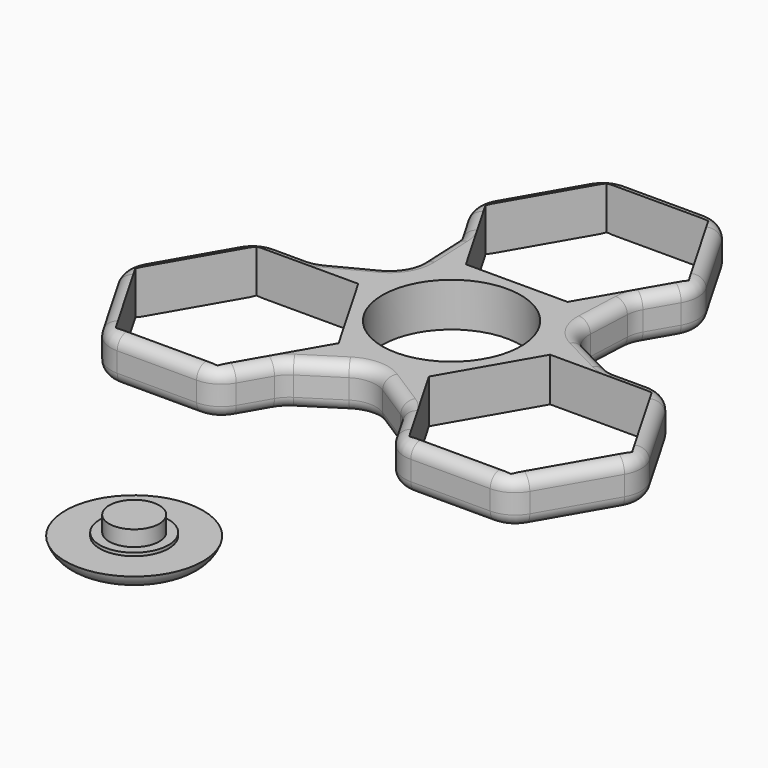
from build123d import *

# Parameters (mm, degrees)
F1_DEPTH       = 7
F2_R           = 5
F3_COUNT       = 3
F4_R           = 5
F5_R           = 11
F5_R_2         = 5.5
F6_DEPTH       = 2.5
F5_R_3         = 4
F7_DEPTH       = 3
F8_DEPTH       = 5.5
F10_T1_DEPTH   = 6.9965201323
F10_T3_DEPTH   = 6.9864388907
F10_T5_DEPTH   = 6.9965201323
F10_T7_DEPTH   = 5.1304731345
F10_T9_DEPTH   = 5.1287182285
F10_T11_DEPTH  = 12.7017059222
F10_T13_DEPTH  = 12.7017059222
F10_T15_DEPTH  = 12.7017059222
F10_T17_DEPTH  = 12.7017059222
F10_T19_DEPTH  = 12.7017059222
F10_T21_DEPTH  = 12.7017059222
F10_T23_DEPTH  = 5.1287182285
F10_T25_DEPTH  = 5.1304731345
F10_T27_DEPTH  = 6.9965201323
F10_T29_DEPTH  = 6.9864388907
F10_T31_DEPTH  = 6.9864388907
F10_T33_DEPTH  = 5.1304731345
F10_T35_DEPTH  = 5.1287182285
F10_T37_DEPTH  = 12.7017059222
F10_T39_DEPTH  = 12.7017059222
F10_T41_DEPTH  = 12.7017059222
F10_T44_ANGLE  = 65.096666036
F10_T46_ANGLE  = 27.4326894179
F10_T48_ANGLE  = 27.4706445461
F10_T50_ANGLE  = 60
F10_T52_ANGLE  = 60
F10_T54_ANGLE  = 60
F10_T56_ANGLE  = 60
F10_T58_ANGLE  = 60
F10_T60_ANGLE  = 60
F10_T62_ANGLE  = 60
F10_T64_ANGLE  = 60
F10_T66_ANGLE  = 27.4706445461
F10_T68_ANGLE  = 27.4326894179
F10_T70_ANGLE  = 65.096666036
F10_T72_ANGLE  = 65.096666036
F10_T74_ANGLE  = 27.4326894179
F10_T76_ANGLE  = 27.4706445461
F10_T78_ANGLE  = 60
F10_T80_ANGLE  = 60
F10_T82_ANGLE  = 60
F10_T84_ANGLE  = 60
F10_T86_ANGLE  = 65.096666036
F10_T88_ANGLE  = 27.4326894179
F10_T90_ANGLE  = 27.4706445461
F10_T92_ANGLE  = 60
F10_T94_ANGLE  = 60
F10_T96_ANGLE  = 60
F10_T98_ANGLE  = 60
F10_T100_ANGLE = 60
F10_T102_ANGLE = 60
F10_T104_ANGLE = 60
F10_T106_ANGLE = 60
F10_T108_ANGLE = 27.4706445461
F10_T110_ANGLE = 27.4326894179
F10_T112_ANGLE = 65.096666036
F10_T114_ANGLE = 65.096666036
F10_T116_ANGLE = 27.4326894179
F10_T118_ANGLE = 27.4706445461
F10_T120_ANGLE = 60
F10_T122_ANGLE = 60
F10_T124_ANGLE = 60
F10_T126_ANGLE = 60


# Not quite as in the source:
# - a fillet or chamfer that OpenCascade refuses, or shapes differently, is made with other operations: its cross-section is extruded or revolved along the edge and cut away or added


with BuildPart() as f1:
    # F0 (on Top) → F1 (new body)
    with BuildSketch(Plane.XY):
        with BuildLine():
            Line((13, 0), (11.075, 0))
            ThreePointArc((11.075, 0), (0, -11.075), (-11.075, 0))
            Line((-11.075, 0), (-13, 0))
            ThreePointArc((-13, 0), (0, -13), (13, 0))
        make_face()
        with BuildLine():
            ThreePointArc((-11.075, 0), (0, 11.075), (11.075, 0))
            Line((11.075, 0), (13, 0))
            ThreePointArc((13, 0), (11.3350959698, 6.3651865139), (6.7668308683, 11.1))
            Line((6.7668308683, 11.1), (-6.7668308683, 11.1))
            ThreePointArc((-6.7668308683, 11.1), (-11.3350959698, 6.3651865139), (-13, 0))
            Line((-13, 0), (-11.075, 0))
        make_face()
        with BuildLine():
            ThreePointArc((6.7668308683, 11.1), (11.3350959698, 6.3651865139), (13, 0))
            Line((13, 0), (13.0126777041, 0))
            Line((13.0126777041, 0), (13.8564064606, 19.1))
            Line((13.8564064606, 19.1), (9.237604307, 11.1))
            Line((9.237604307, 11.1), (6.7668308683, 11.1))
        make_face()
        with BuildLine():
            Line((-13.8564064606, 19.1), (-13, 0))
            ThreePointArc((-13, 0), (-11.3350959698, 6.3651865139), (-6.7668308683, 11.1))
            Line((-6.7668308683, 11.1), (-9.237604307, 11.1))
            Line((-9.237604307, 11.1), (-13.8564064606, 19.1))
        make_face()
        with BuildLine():
            ThreePointArc((-6.7668308683, 11.1), (0, 13), (6.7668308683, 11.1))
            Line((6.7668308683, 11.1), (9.237604307, 11.1))
            Line((9.237604307, 11.1), (13.8564064606, 19.1))
            Line((13.8564064606, 19.1), (18.4752086141, 27.1))
            Line((18.4752086141, 27.1), (9.237604307, 43.1))
            Line((9.237604307, 43.1), (-9.237604307, 43.1))
            Line((-9.237604307, 43.1), (-18.4752086141, 27.1))
            Line((-18.4752086141, 27.1), (-13.8564064606, 19.1))
            Line((-13.8564064606, 19.1), (-9.237604307, 11.1))
            Line((-9.237604307, 11.1), (-6.7668308683, 11.1))
        make_face()
        Polygon((16.2524100777, 27.1), (8.1262050388, 13.025), (-8.1262050388, 13.025), (-16.2524100777, 27.1), (-11.1141951775, 35.9996492673), (-8.1262050388, 41.175), (8.1262050388, 41.175), (11.1141951775, 35.9996492673), align=None, mode=Mode.SUBTRACT)
        with BuildLine():
            Line((-6.7668308683, 11.1), (6.7668308683, 11.1))
            ThreePointArc((6.7668308683, 11.1), (0, 13), (-6.7668308683, 11.1))
        make_face()
    extrude(amount=F1_DEPTH)

    # F2
    f2_edges = [f1.edges().sort_by_distance(p)[0] for p in [
        (-18.475209, 27.1, 3.5),
        (-9.237604, 43.1, 3.5),
        (9.237604, 43.1, 3.5),
        (18.475209, 27.1, 3.5),
        (13.856406, 19.1, 3.5),
        (-13.856406, 19.1, 3.5),
    ]]
    fillet(f2_edges, radius=F2_R)

    # F3: F1 ×3 about axis
    f3_axis = Axis((0, 0, 0), (0, 0, -1))


with BuildPart() as f1_1:
    add(f1.part)
    for i in range(1, F3_COUNT):
        add(f1.part.rotate(f3_axis, i * 360 / F3_COUNT))

    # F4
    f4_edges = [f1_1.edges().sort_by_distance(p)[0] for p in [
        (-13.345851, 7.713337, 3.5),
        (13.352872, 7.701177, 3.5),
        (-0.007021, -15.414515, 3.5),
    ]]
    fillet(f4_edges, radius=F4_R)

    # F10: fillet of radius 1.925 on 84 edges, made by hand

    # F10_s2 → F10_t1 (cut)
    with BuildSketch(Plane(origin=(0.5063723559, 11.4630583874, 0), x_dir=(0, 0, 1), z_dir=(0.0441312433, 0.9990257421, 0))):
        with BuildLine():
            ThreePointArc((5.075, 13), (6.4361805538, 12.4361805538), (7, 11.075))
            Line((7, 11.075), (7, 13))
            Line((7, 13), (5.075, 13))
        make_face()
        with BuildLine():
            ThreePointArc((0, 11.075), (0.5638194462, 12.4361805538), (1.925, 13))
            Line((1.925, 13), (0, 13))
            Line((0, 13), (0, 11.075))
        make_face()
    extrude(amount=F10_T1_DEPTH, mode=Mode.SUBTRACT)

    # F10_s4 → F10_t3 (cut)
    with BuildSketch(Plane(origin=(-15.5751419663, -9.9482027869, 0), x_dir=(0, 0, 1), z_dir=(0.8427596491, 0.5382900463, 0))):
        with BuildLine():
            ThreePointArc((0, 11.0619517506), (0.5638194462, 12.4231323044), (1.925, 12.9869517506))
            Line((1.925, 12.9869517506), (0, 12.9869517506))
            Line((0, 12.9869517506), (0, 11.0619517506))
        make_face()
        with BuildLine():
            ThreePointArc((5.075, 12.9869517506), (6.4361805538, 12.4231323044), (7, 11.0619517506))
            Line((7, 11.0619517506), (7, 12.9869517506))
            Line((7, 12.9869517506), (5.075, 12.9869517506))
        make_face()
    extrude(amount=F10_T3_DEPTH, mode=Mode.SUBTRACT)

    # F10_s6 → F10_t5 (cut)
    with BuildSketch(Plane(origin=(9.6741135906, -6.1700605177, 0), x_dir=(0, 0, 1), z_dir=(0.84311605, -0.5377316488, 0))):
        with BuildLine():
            ThreePointArc((0, 11.075), (0.5638194462, 12.4361805538), (1.925, 13))
            Line((1.925, 13), (0, 13))
            Line((0, 13), (0, 11.075))
        make_face()
        with BuildLine():
            ThreePointArc((5.075, 13), (6.4361805538, 12.4361805538), (7, 11.075))
            Line((7, 11.075), (7, 13))
            Line((7, 13), (5.075, 13))
        make_face()
    extrude(amount=F10_T5_DEPTH, mode=Mode.SUBTRACT)

    # F10_s8 → F10_t7 (cut)
    with BuildSketch(Plane(origin=(-14.9100707018, -25.825, 0), x_dir=(0, 0, 1), z_dir=(0.5, 0.8660254038, 0))):
        with BuildLine():
            ThreePointArc((0, 0.525), (0.5638194462, 1.8861805538), (1.925, 2.45))
            Line((1.925, 2.45), (0, 2.45))
            Line((0, 2.45), (0, 0.525))
        make_face()
        with BuildLine():
            ThreePointArc((5.075, 2.45), (6.4361805538, 1.8861805538), (7, 0.525))
            Line((7, 0.525), (7, 2.45))
            Line((7, 2.45), (5.075, 2.45))
        make_face()
    extrude(amount=F10_T7_DEPTH, mode=Mode.SUBTRACT)

    # F10_s10 → F10_t9 (cut)
    with BuildSketch(Plane(origin=(12.3457115876, -21.3833997253, 0), x_dir=(0, 0, 1), z_dir=(0.5, -0.8660254038, 0))):
        with BuildLine():
            ThreePointArc((0, 0.525), (0.5638194462, 1.8861805538), (1.925, 2.45))
            Line((1.925, 2.45), (0, 2.45))
            Line((0, 2.45), (0, 0.525))
        make_face()
        with BuildLine():
            ThreePointArc((5.075, 2.45), (6.4361805538, 1.8861805538), (7, 0.525))
            Line((7, 0.525), (7, 2.45))
            Line((7, 2.45), (5.075, 2.45))
        make_face()
    extrude(amount=F10_T9_DEPTH, mode=Mode.SUBTRACT)

    # F10_s12 → F10_t11 (cut)
    with BuildSketch(Plane.YZ.offset(-29.8201414036)):
        with BuildLine():
            ThreePointArc((-27.625, 0), (-28.9861805538, 0.5638194462), (-29.55, 1.925))
            Line((-29.55, 1.925), (-29.55, 0))
            Line((-29.55, 0), (-27.625, 0))
        make_face()
        with BuildLine():
            ThreePointArc((-29.55, 5.075), (-28.9861805538, 6.4361805538), (-27.625, 7))
            Line((-27.625, 7), (-29.55, 7))
            Line((-29.55, 7), (-29.55, 5.075))
        make_face()
    extrude(amount=F10_T11_DEPTH, mode=Mode.SUBTRACT)

    # F10_s14 → F10_t13 (cut)
    with BuildSketch(Plane.YZ.offset(17.1184354815)):
        with BuildLine():
            ThreePointArc((-27.625, 0), (-28.9861805538, 0.5638194462), (-29.55, 1.925))
            Line((-29.55, 1.925), (-29.55, 0))
            Line((-29.55, 0), (-27.625, 0))
        make_face()
        with BuildLine():
            ThreePointArc((-29.55, 5.075), (-28.9861805538, 6.4361805538), (-27.625, 7))
            Line((-27.625, 7), (-29.55, 7))
            Line((-29.55, 7), (-29.55, 5.075))
        make_face()
    extrude(amount=F10_T13_DEPTH, mode=Mode.SUBTRACT)

    # F10_s16 → F10_t15 (cut)
    with BuildSketch(Plane(origin=(-3.1754264805, 5.5, 0), x_dir=(0, 0, 1), z_dir=(0.5, -0.8660254038, 0))):
        with BuildLine():
            ThreePointArc((0, 41.175), (0.5638194462, 42.5361805538), (1.925, 43.1))
            Line((1.925, 43.1), (0, 43.1))
            Line((0, 43.1), (0, 41.175))
        make_face()
        with BuildLine():
            ThreePointArc((5.075, 43.1), (6.4361805538, 42.5361805538), (7, 41.175))
            Line((7, 41.175), (7, 43.1))
            Line((7, 43.1), (5.075, 43.1))
        make_face()
    extrude(amount=F10_T15_DEPTH, mode=Mode.SUBTRACT)

    # F10_s18 → F10_t17 (cut)
    with BuildSketch(Plane(origin=(-3.1754264805, -5.5, 0), x_dir=(0, 0, 1), z_dir=(0.5, 0.8660254038, 0))):
        with BuildLine():
            ThreePointArc((0, 41.175), (0.5638194462, 42.5361805538), (1.925, 43.1))
            Line((1.925, 43.1), (0, 43.1))
            Line((0, 43.1), (0, 41.175))
        make_face()
        with BuildLine():
            ThreePointArc((5.075, 43.1), (6.4361805538, 42.5361805538), (7, 41.175))
            Line((7, 41.175), (7, 43.1))
            Line((7, 43.1), (5.075, 43.1))
        make_face()
    extrude(amount=F10_T17_DEPTH, mode=Mode.SUBTRACT)

    # F10_s20 → F10_t19 (cut)
    with BuildSketch(Plane(origin=(-8.5592177407, -14.825, 0), x_dir=(0, 0, 1), z_dir=(-0.5, -0.8660254038, 0))):
        with BuildLine():
            ThreePointArc((0, 27.625), (0.5638194462, 28.9861805538), (1.925, 29.55))
            Line((1.925, 29.55), (0, 29.55))
            Line((0, 29.55), (0, 27.625))
        make_face()
        with BuildLine():
            ThreePointArc((5.075, 29.55), (6.4361805538, 28.9861805538), (7, 27.625))
            Line((7, 27.625), (7, 29.55))
            Line((7, 29.55), (5.075, 29.55))
        make_face()
    extrude(amount=F10_T19_DEPTH, mode=Mode.SUBTRACT)

    # F10_s22 → F10_t21 (cut)
    with BuildSketch(Plane(origin=(14.9100707018, -25.825, 0), x_dir=(0, 0, 1), z_dir=(-0.5, 0.8660254038, 0))):
        with BuildLine():
            ThreePointArc((0, 27.625), (0.5638194462, 28.9861805538), (1.925, 29.55))
            Line((1.925, 29.55), (0, 29.55))
            Line((0, 29.55), (0, 27.625))
        make_face()
        with BuildLine():
            ThreePointArc((5.075, 29.55), (6.4361805538, 28.9861805538), (7, 27.625))
            Line((7, 27.625), (7, 29.55))
            Line((7, 29.55), (5.075, 29.55))
        make_face()
    extrude(amount=F10_T21_DEPTH, mode=Mode.SUBTRACT)

    # F10_s24 → F10_t23 (cut)
    with BuildSketch(Plane.YZ.offset(-29.8201414036)):
        with BuildLine():
            ThreePointArc((0.525, 0), (1.8861805538, 0.5638194462), (2.45, 1.925))
            Line((2.45, 1.925), (2.45, 0))
            Line((2.45, 0), (0.525, 0))
        make_face()
        with BuildLine():
            ThreePointArc((2.45, 5.075), (1.8861805538, 6.4361805538), (0.525, 7))
            Line((0.525, 7), (2.45, 7))
            Line((2.45, 7), (2.45, 5.075))
        make_face()
    extrude(amount=F10_T23_DEPTH, mode=Mode.SUBTRACT)

    # F10_s26 → F10_t25 (cut)
    with BuildSketch(Plane.YZ.offset(24.6896682691)):
        with BuildLine():
            ThreePointArc((0.525, 0), (1.8861805538, 0.5638194462), (2.45, 1.925))
            Line((2.45, 1.925), (2.45, 0))
            Line((2.45, 0), (0.525, 0))
        make_face()
        with BuildLine():
            ThreePointArc((2.45, 5.075), (1.8861805538, 6.4361805538), (0.525, 7))
            Line((0.525, 7), (2.45, 7))
            Line((2.45, 7), (2.45, 5.075))
        make_face()
    extrude(amount=F10_T25_DEPTH, mode=Mode.SUBTRACT)

    # F10_s28 → F10_t27 (cut)
    with BuildSketch(Plane(origin=(-10.1804859465, -5.2929978697, 0), x_dir=(0, 0, 1), z_dir=(-0.8872472933, -0.4612940932, 0))):
        with BuildLine():
            ThreePointArc((0, 11.075), (0.5638194462, 12.4361805538), (1.925, 13))
            Line((1.925, 13), (0, 13))
            Line((0, 13), (0, 11.075))
        make_face()
        with BuildLine():
            ThreePointArc((5.075, 13), (6.4361805538, 12.4361805538), (7, 11.075))
            Line((7, 11.075), (7, 13))
            Line((7, 13), (5.075, 13))
        make_face()
    extrude(amount=F10_T27_DEPTH, mode=Mode.SUBTRACT)

    # F10_s30 → F10_t29 (cut)
    with BuildSketch(Plane(origin=(16.4029673186, -8.5143672169, 0), x_dir=(0, 0, 1), z_dir=(-0.8875526792, 0.4607062422, 0))):
        with BuildLine():
            ThreePointArc((0, 11.0619517506), (0.5638194462, 12.4231323044), (1.925, 12.9869517506))
            Line((1.925, 12.9869517506), (0, 12.9869517506))
            Line((0, 12.9869517506), (0, 11.0619517506))
        make_face()
        with BuildLine():
            ThreePointArc((5.075, 12.9869517506), (6.4361805538, 12.4231323044), (7, 11.0619517506))
            Line((7, 11.0619517506), (7, 12.9869517506))
            Line((7, 12.9869517506), (5.075, 12.9869517506))
        make_face()
    extrude(amount=F10_T29_DEPTH, mode=Mode.SUBTRACT)

    # F10_s32 → F10_t31 (cut)
    with BuildSketch(Plane(origin=(-0.8278253523, 18.4625700038, 0), x_dir=(0, 0, 1), z_dir=(0.0447930301, -0.9989962885, 0))):
        with BuildLine():
            ThreePointArc((0, 11.0619517506), (0.5638194462, 12.4231323044), (1.925, 12.9869517506))
            Line((1.925, 12.9869517506), (0, 12.9869517506))
            Line((0, 12.9869517506), (0, 11.0619517506))
        make_face()
        with BuildLine():
            ThreePointArc((5.075, 12.9869517506), (6.4361805538, 12.4231323044), (7, 11.0619517506))
            Line((7, 11.0619517506), (7, 12.9869517506))
            Line((7, 12.9869517506), (5.075, 12.9869517506))
        make_face()
    extrude(amount=F10_T31_DEPTH, mode=Mode.SUBTRACT)

    # F10_s34 → F10_t33 (cut)
    with BuildSketch(Plane(origin=(-14.9100707018, 25.825, 0), x_dir=(0, 0, 1), z_dir=(0.5, -0.8660254038, 0))):
        with BuildLine():
            ThreePointArc((0, 0.525), (0.5638194462, 1.8861805538), (1.925, 2.45))
            Line((1.925, 2.45), (0, 2.45))
            Line((0, 2.45), (0, 0.525))
        make_face()
        with BuildLine():
            ThreePointArc((5.075, 2.45), (6.4361805538, 1.8861805538), (7, 0.525))
            Line((7, 0.525), (7, 2.45))
            Line((7, 2.45), (5.075, 2.45))
        make_face()
    extrude(amount=F10_T33_DEPTH, mode=Mode.SUBTRACT)

    # F10_s36 → F10_t35 (cut)
    with BuildSketch(Plane(origin=(12.3457115876, 21.3833997253, 0), x_dir=(0, 0, 1), z_dir=(0.5, 0.8660254038, 0))):
        with BuildLine():
            ThreePointArc((0, 0.525), (0.5638194462, 1.8861805538), (1.925, 2.45))
            Line((1.925, 2.45), (0, 2.45))
            Line((0, 2.45), (0, 0.525))
        make_face()
        with BuildLine():
            ThreePointArc((5.075, 2.45), (6.4361805538, 1.8861805538), (7, 0.525))
            Line((7, 0.525), (7, 2.45))
            Line((7, 2.45), (5.075, 2.45))
        make_face()
    extrude(amount=F10_T35_DEPTH, mode=Mode.SUBTRACT)

    # F10_s38 → F10_t37 (cut)
    with BuildSketch(Plane(origin=(14.9100707018, 25.825, 0), x_dir=(0, 0, 1), z_dir=(-0.5, -0.8660254038, 0))):
        with BuildLine():
            ThreePointArc((0, 27.625), (0.5638194462, 28.9861805538), (1.925, 29.55))
            Line((1.925, 29.55), (0, 29.55))
            Line((0, 29.55), (0, 27.625))
        make_face()
        with BuildLine():
            ThreePointArc((5.075, 29.55), (6.4361805538, 28.9861805538), (7, 27.625))
            Line((7, 27.625), (7, 29.55))
            Line((7, 29.55), (5.075, 29.55))
        make_face()
    extrude(amount=F10_T37_DEPTH, mode=Mode.SUBTRACT)

    # F10_s40 → F10_t39 (cut)
    with BuildSketch(Plane(origin=(-8.5592177407, 14.825, 0), x_dir=(0, 0, 1), z_dir=(-0.5, 0.8660254038, 0))):
        with BuildLine():
            ThreePointArc((0, 27.625), (0.5638194462, 28.9861805538), (1.925, 29.55))
            Line((1.925, 29.55), (0, 29.55))
            Line((0, 29.55), (0, 27.625))
        make_face()
        with BuildLine():
            ThreePointArc((5.075, 29.55), (6.4361805538, 28.9861805538), (7, 27.625))
            Line((7, 27.625), (7, 29.55))
            Line((7, 29.55), (5.075, 29.55))
        make_face()
    extrude(amount=F10_T39_DEPTH, mode=Mode.SUBTRACT)

    # F10_s42 → F10_t41 (cut)
    with BuildSketch(Plane.YZ.offset(-6.3508529611)):
        with BuildLine():
            ThreePointArc((41.175, 0), (42.5361805538, 0.5638194462), (43.1, 1.925))
            Line((43.1, 1.925), (43.1, 0))
            Line((43.1, 0), (41.175, 0))
        make_face()
        with BuildLine():
            ThreePointArc((43.1, 5.075), (42.5361805538, 6.4361805538), (41.175, 7))
            Line((41.175, 7), (43.1, 7))
            Line((43.1, 7), (43.1, 5.075))
        make_face()
    extrude(amount=F10_T41_DEPTH, mode=Mode.SUBTRACT)

    # F10_s43 → F10_t44 (revolve, cut)
    with BuildSketch(Plane(origin=(9.6741135906, -6.1700605177, 0), x_dir=(0, 0, 1), z_dir=(0.84311605, -0.5377316488, 0))):
        with BuildLine():
            ThreePointArc((0, 11.075), (0.5638194462, 12.4361805538), (1.925, 13))
            Line((1.925, 13), (0, 13))
            Line((0, 13), (0, 11.075))
        make_face()
    revolve(axis=Axis((-0.0050560886, -21.3461494184, 0), (0, 0, 1)), revolution_arc=F10_T44_ANGLE, mode=Mode.SUBTRACT)

    # F10_s45 → F10_t46 (revolve, cut)
    with BuildSketch(Plane(origin=(-12.3448341345, -21.3818799321, 0), x_dir=(0, 0, 1), z_dir=(-0.5, -0.8660254038, 0))):
        with BuildLine():
            ThreePointArc((0, -0.525), (0.5638194462, -1.8861805538), (1.925, -2.45))
            Line((1.925, -2.45), (0, -2.45))
            Line((0, -2.45), (0, -0.525))
        make_face()
    revolve(axis=Axis((-5.8929448764, -25.1068799321, 0), (0, 0, -1)), revolution_arc=F10_T46_ANGLE, mode=Mode.SUBTRACT)

    # F10_s47 → F10_t48 (revolve, cut)
    with BuildSketch(Plane(origin=(15.5729920086, -9.9323108246, 0), x_dir=(0, 0, 1), z_dir=(-0.84311605, 0.5377316488, 0))):
        with BuildLine():
            ThreePointArc((0, -11.075), (0.5638194462, -12.4361805538), (1.925, -13))
            Line((1.925, -13), (0, -13))
            Line((0, -13), (0, -11.075))
        make_face()
    revolve(axis=Axis((5.8938223294, -25.1083997253, 0), (0, 0, -1)), revolution_arc=F10_T48_ANGLE, mode=Mode.SUBTRACT)

    # F10_s49 → F10_t50 (revolve, cut)
    with BuildSketch(Plane.YZ.offset(-17.1184354815)):
        with BuildLine():
            ThreePointArc((-27.625, 0), (-28.9861805538, 0.5638194462), (-29.55, 1.925))
            Line((-29.55, 1.925), (-29.55, 0))
            Line((-29.55, 0), (-27.625, 0))
        make_face()
    revolve(axis=Axis((-17.1184354815, -24.55, 0), (0, 0, 1)), revolution_arc=F10_T50_ANGLE, mode=Mode.SUBTRACT)

    # F10_s51 → F10_t52 (revolve, cut)
    with BuildSketch(Plane(origin=(14.9100707018, -25.825, 0), x_dir=(0, 0, 1), z_dir=(-0.5, 0.8660254038, 0))):
        with BuildLine():
            ThreePointArc((0, -0.525), (0.5638194462, -1.8861805538), (1.925, -2.45))
            Line((1.925, -2.45), (0, -2.45))
            Line((0, -2.45), (0, -0.525))
        make_face()
    revolve(axis=Axis((17.1184354815, -24.55, 0), (0, 0, 1)), revolution_arc=F10_T52_ANGLE, mode=Mode.SUBTRACT)

    # F10_s53 → F10_t54 (revolve, cut)
    with BuildSketch(Plane(origin=(3.1754264805, -5.5, 0), x_dir=(0, 0, 1), z_dir=(-0.5, 0.8660254038, 0))):
        with BuildLine():
            ThreePointArc((0, -41.175), (0.5638194462, -42.5361805538), (1.925, -43.1))
            Line((1.925, -43.1), (0, -43.1))
            Line((0, -43.1), (0, -41.175))
        make_face()
    revolve(axis=Axis((-29.8201414036, -24.55, 0), (0, 0, 1)), revolution_arc=F10_T54_ANGLE, mode=Mode.SUBTRACT)

    # F10_s55 → F10_t56 (revolve, cut)
    with BuildSketch(Plane.YZ.offset(29.8201414036)):
        with BuildLine():
            ThreePointArc((-27.625, 0), (-28.9861805538, 0.5638194462), (-29.55, 1.925))
            Line((-29.55, 1.925), (-29.55, 0))
            Line((-29.55, 0), (-27.625, 0))
        make_face()
    revolve(axis=Axis((29.8201414036, -24.55, 0), (0, 0, 1)), revolution_arc=F10_T56_ANGLE, mode=Mode.SUBTRACT)

    # F10_s57 → F10_t58 (revolve, cut)
    with BuildSketch(Plane(origin=(-14.9100707018, -25.825, 0), x_dir=(0, 0, 1), z_dir=(0.5, 0.8660254038, 0))):
        with BuildLine():
            ThreePointArc((0, -27.625), (0.5638194462, -28.9861805538), (1.925, -29.55))
            Line((1.925, -29.55), (0, -29.55))
            Line((0, -29.55), (0, -27.625))
        make_face()
    revolve(axis=Axis((-36.1709943647, -13.55, 0), (0, 0, 1)), revolution_arc=F10_T58_ANGLE, mode=Mode.SUBTRACT)

    # F10_s59 → F10_t60 (revolve, cut)
    with BuildSketch(Plane(origin=(3.1754264805, 5.5, 0), x_dir=(0, 0, 1), z_dir=(-0.5, -0.8660254038, 0))):
        with BuildLine():
            ThreePointArc((0, -41.175), (0.5638194462, -42.5361805538), (1.925, -43.1))
            Line((1.925, -43.1), (0, -43.1))
            Line((0, -43.1), (0, -41.175))
        make_face()
    revolve(axis=Axis((36.1709943647, -13.55, 0), (0, 0, 1)), revolution_arc=F10_T60_ANGLE, mode=Mode.SUBTRACT)

    # F10_s61 → F10_t62 (revolve, cut)
    with BuildSketch(Plane.YZ.offset(-29.8201414036)):
        with BuildLine():
            ThreePointArc((0.525, 0), (1.8861805538, 0.5638194462), (2.45, 1.925))
            Line((2.45, 1.925), (2.45, 0))
            Line((2.45, 0), (0.525, 0))
        make_face()
    revolve(axis=Axis((-29.8201414036, -2.55, 0), (0, 0, 1)), revolution_arc=F10_T62_ANGLE, mode=Mode.SUBTRACT)

    # F10_s63 → F10_t64 (revolve, cut)
    with BuildSketch(Plane(origin=(8.5592177407, -14.825, 0), x_dir=(0, 0, 1), z_dir=(0.5, -0.8660254038, 0))):
        with BuildLine():
            ThreePointArc((0, -27.625), (0.5638194462, -28.9861805538), (1.925, -29.55))
            Line((1.925, -29.55), (0, -29.55))
            Line((0, -29.55), (0, -27.625))
        make_face()
    revolve(axis=Axis((29.8201414036, -2.55, 0), (0, 0, 1)), revolution_arc=F10_T64_ANGLE, mode=Mode.SUBTRACT)

    # F10_s65 → F10_t66 (revolve, cut)
    with BuildSketch(Plane(origin=(-16.3881294967, -8.5204512801, 0), x_dir=(0, 0, 1), z_dir=(0.8872472933, 0.4612940932, 0))):
        with BuildLine():
            ThreePointArc((0, -11.075), (0.5638194462, -12.4361805538), (1.925, -13))
            Line((1.925, -13), (0, -13))
            Line((0, -13), (0, -11.075))
        make_face()
    revolve(axis=Axis((-24.6914231752, 7.45, 0), (0, 0, -1)), revolution_arc=F10_T66_ANGLE, mode=Mode.SUBTRACT)

    # F10_s67 → F10_t68 (revolve, cut)
    with BuildSketch(Plane.YZ.offset(24.6896682691)):
        with BuildLine():
            ThreePointArc((0.525, 0), (1.8861805538, 0.5638194462), (2.45, 1.925))
            Line((2.45, 1.925), (2.45, 0))
            Line((2.45, 0), (0.525, 0))
        make_face()
    revolve(axis=Axis((24.6896682691, 7.45, 0), (0, 0, -1)), revolution_arc=F10_T68_ANGLE, mode=Mode.SUBTRACT)

    # F10_s69 → F10_t70 (revolve, cut)
    with BuildSketch(Plane(origin=(-10.1804859465, -5.2929978697, 0), x_dir=(0, 0, 1), z_dir=(-0.8872472933, -0.4612940932, 0))):
        with BuildLine():
            ThreePointArc((0, 11.075), (0.5638194462, 12.4361805538), (1.925, 13))
            Line((1.925, 13), (0, 13))
            Line((0, 13), (0, 11.075))
        make_face()
    revolve(axis=Axis((-18.483779625, 10.6774534104, 0), (0, 0, 1)), revolution_arc=F10_T70_ANGLE, mode=Mode.SUBTRACT)

    # F10_s71 → F10_t72 (revolve, cut)
    with BuildSketch(Plane(origin=(0.5063723559, 11.4630583874, 0), x_dir=(0, 0, 1), z_dir=(0.0441312433, 0.9990257421, 0))):
        with BuildLine():
            ThreePointArc((0, 11.075), (0.5638194462, 12.4361805538), (1.925, 13))
            Line((1.925, 13), (0, 13))
            Line((0, 13), (0, 11.075))
        make_face()
    revolve(axis=Axis((18.4888357136, 10.668696008, 0), (0, 0, 1)), revolution_arc=F10_T72_ANGLE, mode=Mode.SUBTRACT)

    # F10_s73 → F10_t74 (revolve, cut)
    with BuildSketch(Plane(origin=(-12.3448341345, 21.3818799321, 0), x_dir=(0, 0, 1), z_dir=(-0.5, 0.8660254038, 0))):
        with BuildLine():
            ThreePointArc((0, -0.525), (0.5638194462, -1.8861805538), (1.925, -2.45))
            Line((1.925, -2.45), (0, -2.45))
            Line((0, -2.45), (0, -0.525))
        make_face()
    revolve(axis=Axis((-18.7967233927, 17.6568799321, 0), (0, 0, -1)), revolution_arc=F10_T74_ANGLE, mode=Mode.SUBTRACT)

    # F10_s75 → F10_t76 (revolve, cut)
    with BuildSketch(Plane(origin=(0.8151374881, 18.4527621047, 0), x_dir=(0, 0, 1), z_dir=(-0.0441312433, -0.9990257421, 0))):
        with BuildLine():
            ThreePointArc((0, -11.075), (0.5638194462, -12.4361805538), (1.925, -13))
            Line((1.925, -13), (0, -13))
            Line((0, -13), (0, -11.075))
        make_face()
    revolve(axis=Axis((18.7976008458, 17.6583997253, 0), (0, 0, -1)), revolution_arc=F10_T76_ANGLE, mode=Mode.SUBTRACT)

    # F10_s77 → F10_t78 (revolve, cut)
    with BuildSketch(Plane(origin=(8.5592177407, 14.825, 0), x_dir=(0, 0, 1), z_dir=(0.5, 0.8660254038, 0))):
        with BuildLine():
            ThreePointArc((0, -27.625), (0.5638194462, -28.9861805538), (1.925, -29.55))
            Line((1.925, -29.55), (0, -29.55))
            Line((0, -29.55), (0, -27.625))
        make_face()
    revolve(axis=Axis((-12.7017059222, 27.1, 0), (0, 0, 1)), revolution_arc=F10_T78_ANGLE, mode=Mode.SUBTRACT)

    # F10_s79 → F10_t80 (revolve, cut)
    with BuildSketch(Plane(origin=(14.9100707018, 25.825, 0), x_dir=(0, 0, 1), z_dir=(-0.5, -0.8660254038, 0))):
        with BuildLine():
            ThreePointArc((0, -0.525), (0.5638194462, -1.8861805538), (1.925, -2.45))
            Line((1.925, -2.45), (0, -2.45))
            Line((0, -2.45), (0, -0.525))
        make_face()
    revolve(axis=Axis((12.7017059222, 27.1, 0), (0, 0, 1)), revolution_arc=F10_T80_ANGLE, mode=Mode.SUBTRACT)

    # F10_s81 → F10_t82 (revolve, cut)
    with BuildSketch(Plane.YZ.offset(-6.3508529611)):
        with BuildLine():
            ThreePointArc((41.175, 0), (42.5361805538, 0.5638194462), (43.1, 1.925))
            Line((43.1, 1.925), (43.1, 0))
            Line((43.1, 0), (41.175, 0))
        make_face()
    revolve(axis=Axis((-6.3508529611, 38.1, 0), (0, 0, 1)), revolution_arc=F10_T82_ANGLE, mode=Mode.SUBTRACT)

    # F10_s83 → F10_t84 (revolve, cut)
    with BuildSketch(Plane(origin=(-14.9100707018, 25.825, 0), x_dir=(0, 0, 1), z_dir=(0.5, -0.8660254038, 0))):
        with BuildLine():
            ThreePointArc((0, -27.625), (0.5638194462, -28.9861805538), (1.925, -29.55))
            Line((1.925, -29.55), (0, -29.55))
            Line((0, -29.55), (0, -27.625))
        make_face()
    revolve(axis=Axis((6.3508529611, 38.1, 0), (0, 0, 1)), revolution_arc=F10_T84_ANGLE, mode=Mode.SUBTRACT)

    # F10_s85 → F10_t86 (revolve, cut)
    with BuildSketch(Plane(origin=(9.6741135906, -6.1700605177, 0), x_dir=(0, 0, 1), z_dir=(0.84311605, -0.5377316488, 0))):
        with BuildLine():
            ThreePointArc((5.075, 13), (6.4361805538, 12.4361805538), (7, 11.075))
            Line((7, 11.075), (7, 13))
            Line((7, 13), (5.075, 13))
        make_face()
    revolve(axis=Axis((-0.0050560886, -21.3461494184, 7), (0, 0, 1)), revolution_arc=F10_T86_ANGLE, mode=Mode.SUBTRACT)

    # F10_s87 → F10_t88 (revolve, cut)
    with BuildSketch(Plane(origin=(-12.3448341345, -21.3818799321, 0), x_dir=(0, 0, 1), z_dir=(-0.5, -0.8660254038, 0))):
        with BuildLine():
            ThreePointArc((5.075, -2.45), (6.4361805538, -1.8861805538), (7, -0.525))
            Line((7, -0.525), (7, -2.45))
            Line((7, -2.45), (5.075, -2.45))
        make_face()
    revolve(axis=Axis((-5.8929448764, -25.1068799321, 7), (0, 0, -1)), revolution_arc=F10_T88_ANGLE, mode=Mode.SUBTRACT)

    # F10_s89 → F10_t90 (revolve, cut)
    with BuildSketch(Plane(origin=(15.5729920086, -9.9323108246, 0), x_dir=(0, 0, 1), z_dir=(-0.84311605, 0.5377316488, 0))):
        with BuildLine():
            ThreePointArc((5.075, -13), (6.4361805538, -12.4361805538), (7, -11.075))
            Line((7, -11.075), (7, -13))
            Line((7, -13), (5.075, -13))
        make_face()
    revolve(axis=Axis((5.8938223294, -25.1083997253, 7), (0, 0, -1)), revolution_arc=F10_T90_ANGLE, mode=Mode.SUBTRACT)

    # F10_s91 → F10_t92 (revolve, cut)
    with BuildSketch(Plane.YZ.offset(-17.1184354815)):
        with BuildLine():
            ThreePointArc((-29.55, 5.075), (-28.9861805538, 6.4361805538), (-27.625, 7))
            Line((-27.625, 7), (-29.55, 7))
            Line((-29.55, 7), (-29.55, 5.075))
        make_face()
    revolve(axis=Axis((-17.1184354815, -24.55, 7), (0, 0, 1)), revolution_arc=F10_T92_ANGLE, mode=Mode.SUBTRACT)

    # F10_s93 → F10_t94 (revolve, cut)
    with BuildSketch(Plane(origin=(14.9100707018, -25.825, 0), x_dir=(0, 0, 1), z_dir=(-0.5, 0.8660254038, 0))):
        with BuildLine():
            ThreePointArc((5.075, -2.45), (6.4361805538, -1.8861805538), (7, -0.525))
            Line((7, -0.525), (7, -2.45))
            Line((7, -2.45), (5.075, -2.45))
        make_face()
    revolve(axis=Axis((17.1184354815, -24.55, 7), (0, 0, 1)), revolution_arc=F10_T94_ANGLE, mode=Mode.SUBTRACT)

    # F10_s95 → F10_t96 (revolve, cut)
    with BuildSketch(Plane(origin=(3.1754264805, -5.5, 0), x_dir=(0, 0, 1), z_dir=(-0.5, 0.8660254038, 0))):
        with BuildLine():
            ThreePointArc((5.075, -43.1), (6.4361805538, -42.5361805538), (7, -41.175))
            Line((7, -41.175), (7, -43.1))
            Line((7, -43.1), (5.075, -43.1))
        make_face()
    revolve(axis=Axis((-29.8201414036, -24.55, 7), (0, 0, 1)), revolution_arc=F10_T96_ANGLE, mode=Mode.SUBTRACT)

    # F10_s97 → F10_t98 (revolve, cut)
    with BuildSketch(Plane.YZ.offset(29.8201414036)):
        with BuildLine():
            ThreePointArc((-29.55, 5.075), (-28.9861805538, 6.4361805538), (-27.625, 7))
            Line((-27.625, 7), (-29.55, 7))
            Line((-29.55, 7), (-29.55, 5.075))
        make_face()
    revolve(axis=Axis((29.8201414036, -24.55, 7), (0, 0, 1)), revolution_arc=F10_T98_ANGLE, mode=Mode.SUBTRACT)

    # F10_s99 → F10_t100 (revolve, cut)
    with BuildSketch(Plane(origin=(-14.9100707018, -25.825, 0), x_dir=(0, 0, 1), z_dir=(0.5, 0.8660254038, 0))):
        with BuildLine():
            ThreePointArc((5.075, -29.55), (6.4361805538, -28.9861805538), (7, -27.625))
            Line((7, -27.625), (7, -29.55))
            Line((7, -29.55), (5.075, -29.55))
        make_face()
    revolve(axis=Axis((-36.1709943647, -13.55, 7), (0, 0, 1)), revolution_arc=F10_T100_ANGLE, mode=Mode.SUBTRACT)

    # F10_s101 → F10_t102 (revolve, cut)
    with BuildSketch(Plane(origin=(3.1754264805, 5.5, 0), x_dir=(0, 0, 1), z_dir=(-0.5, -0.8660254038, 0))):
        with BuildLine():
            ThreePointArc((5.075, -43.1), (6.4361805538, -42.5361805538), (7, -41.175))
            Line((7, -41.175), (7, -43.1))
            Line((7, -43.1), (5.075, -43.1))
        make_face()
    revolve(axis=Axis((36.1709943647, -13.55, 7), (0, 0, 1)), revolution_arc=F10_T102_ANGLE, mode=Mode.SUBTRACT)

    # F10_s103 → F10_t104 (revolve, cut)
    with BuildSketch(Plane.YZ.offset(-29.8201414036)):
        with BuildLine():
            ThreePointArc((2.45, 5.075), (1.8861805538, 6.4361805538), (0.525, 7))
            Line((0.525, 7), (2.45, 7))
            Line((2.45, 7), (2.45, 5.075))
        make_face()
    revolve(axis=Axis((-29.8201414036, -2.55, 7), (0, 0, 1)), revolution_arc=F10_T104_ANGLE, mode=Mode.SUBTRACT)

    # F10_s105 → F10_t106 (revolve, cut)
    with BuildSketch(Plane(origin=(8.5592177407, -14.825, 0), x_dir=(0, 0, 1), z_dir=(0.5, -0.8660254038, 0))):
        with BuildLine():
            ThreePointArc((5.075, -29.55), (6.4361805538, -28.9861805538), (7, -27.625))
            Line((7, -27.625), (7, -29.55))
            Line((7, -29.55), (5.075, -29.55))
        make_face()
    revolve(axis=Axis((29.8201414036, -2.55, 7), (0, 0, 1)), revolution_arc=F10_T106_ANGLE, mode=Mode.SUBTRACT)

    # F10_s107 → F10_t108 (revolve, cut)
    with BuildSketch(Plane(origin=(-16.3881294967, -8.5204512801, 0), x_dir=(0, 0, 1), z_dir=(0.8872472933, 0.4612940932, 0))):
        with BuildLine():
            ThreePointArc((5.075, -13), (6.4361805538, -12.4361805538), (7, -11.075))
            Line((7, -11.075), (7, -13))
            Line((7, -13), (5.075, -13))
        make_face()
    revolve(axis=Axis((-24.6914231752, 7.45, 7), (0, 0, -1)), revolution_arc=F10_T108_ANGLE, mode=Mode.SUBTRACT)

    # F10_s109 → F10_t110 (revolve, cut)
    with BuildSketch(Plane.YZ.offset(24.6896682691)):
        with BuildLine():
            ThreePointArc((2.45, 5.075), (1.8861805538, 6.4361805538), (0.525, 7))
            Line((0.525, 7), (2.45, 7))
            Line((2.45, 7), (2.45, 5.075))
        make_face()
    revolve(axis=Axis((24.6896682691, 7.45, 7), (0, 0, -1)), revolution_arc=F10_T110_ANGLE, mode=Mode.SUBTRACT)

    # F10_s111 → F10_t112 (revolve, cut)
    with BuildSketch(Plane(origin=(-10.1804859465, -5.2929978697, 0), x_dir=(0, 0, 1), z_dir=(-0.8872472933, -0.4612940932, 0))):
        with BuildLine():
            ThreePointArc((5.075, 13), (6.4361805538, 12.4361805538), (7, 11.075))
            Line((7, 11.075), (7, 13))
            Line((7, 13), (5.075, 13))
        make_face()
    revolve(axis=Axis((-18.483779625, 10.6774534104, 7), (0, 0, 1)), revolution_arc=F10_T112_ANGLE, mode=Mode.SUBTRACT)

    # F10_s113 → F10_t114 (revolve, cut)
    with BuildSketch(Plane(origin=(0.5063723559, 11.4630583874, 0), x_dir=(0, 0, 1), z_dir=(0.0441312433, 0.9990257421, 0))):
        with BuildLine():
            ThreePointArc((5.075, 13), (6.4361805538, 12.4361805538), (7, 11.075))
            Line((7, 11.075), (7, 13))
            Line((7, 13), (5.075, 13))
        make_face()
    revolve(axis=Axis((18.4888357136, 10.668696008, 7), (0, 0, 1)), revolution_arc=F10_T114_ANGLE, mode=Mode.SUBTRACT)

    # F10_s115 → F10_t116 (revolve, cut)
    with BuildSketch(Plane(origin=(-12.3448341345, 21.3818799321, 0), x_dir=(0, 0, 1), z_dir=(-0.5, 0.8660254038, 0))):
        with BuildLine():
            ThreePointArc((5.075, -2.45), (6.4361805538, -1.8861805538), (7, -0.525))
            Line((7, -0.525), (7, -2.45))
            Line((7, -2.45), (5.075, -2.45))
        make_face()
    revolve(axis=Axis((-18.7967233927, 17.6568799321, 7), (0, 0, -1)), revolution_arc=F10_T116_ANGLE, mode=Mode.SUBTRACT)

    # F10_s117 → F10_t118 (revolve, cut)
    with BuildSketch(Plane(origin=(0.8151374881, 18.4527621047, 0), x_dir=(0, 0, 1), z_dir=(-0.0441312433, -0.9990257421, 0))):
        with BuildLine():
            ThreePointArc((5.075, -13), (6.4361805538, -12.4361805538), (7, -11.075))
            Line((7, -11.075), (7, -13))
            Line((7, -13), (5.075, -13))
        make_face()
    revolve(axis=Axis((18.7976008458, 17.6583997253, 7), (0, 0, -1)), revolution_arc=F10_T118_ANGLE, mode=Mode.SUBTRACT)

    # F10_s119 → F10_t120 (revolve, cut)
    with BuildSketch(Plane(origin=(8.5592177407, 14.825, 0), x_dir=(0, 0, 1), z_dir=(0.5, 0.8660254038, 0))):
        with BuildLine():
            ThreePointArc((5.075, -29.55), (6.4361805538, -28.9861805538), (7, -27.625))
            Line((7, -27.625), (7, -29.55))
            Line((7, -29.55), (5.075, -29.55))
        make_face()
    revolve(axis=Axis((-12.7017059222, 27.1, 7), (0, 0, 1)), revolution_arc=F10_T120_ANGLE, mode=Mode.SUBTRACT)

    # F10_s121 → F10_t122 (revolve, cut)
    with BuildSketch(Plane(origin=(14.9100707018, 25.825, 0), x_dir=(0, 0, 1), z_dir=(-0.5, -0.8660254038, 0))):
        with BuildLine():
            ThreePointArc((5.075, -2.45), (6.4361805538, -1.8861805538), (7, -0.525))
            Line((7, -0.525), (7, -2.45))
            Line((7, -2.45), (5.075, -2.45))
        make_face()
    revolve(axis=Axis((12.7017059222, 27.1, 7), (0, 0, 1)), revolution_arc=F10_T122_ANGLE, mode=Mode.SUBTRACT)

    # F10_s123 → F10_t124 (revolve, cut)
    with BuildSketch(Plane.YZ.offset(-6.3508529611)):
        with BuildLine():
            ThreePointArc((43.1, 5.075), (42.5361805538, 6.4361805538), (41.175, 7))
            Line((41.175, 7), (43.1, 7))
            Line((43.1, 7), (43.1, 5.075))
        make_face()
    revolve(axis=Axis((-6.3508529611, 38.1, 7), (0, 0, 1)), revolution_arc=F10_T124_ANGLE, mode=Mode.SUBTRACT)

    # F10_s125 → F10_t126 (revolve, cut)
    with BuildSketch(Plane(origin=(-14.9100707018, 25.825, 0), x_dir=(0, 0, 1), z_dir=(0.5, -0.8660254038, 0))):
        with BuildLine():
            ThreePointArc((5.075, -29.55), (6.4361805538, -28.9861805538), (7, -27.625))
            Line((7, -27.625), (7, -29.55))
            Line((7, -29.55), (5.075, -29.55))
        make_face()
    revolve(axis=Axis((6.3508529611, 38.1, 7), (0, 0, 1)), revolution_arc=F10_T126_ANGLE, mode=Mode.SUBTRACT)


with BuildPart() as f6:
    # F5 (on Top) → F6 (new body)
    with BuildSketch(Plane.XY):
        with Locations((0, -63.4327519663)):
            Circle(F5_R)
        with Locations((0, -63.4327519663)):
            Circle(F5_R_2, mode=Mode.SUBTRACT)
    extrude(amount=F6_DEPTH)

    # F5 (on Top) → F7 (join, through all)
    with BuildSketch(Plane.XY):
        with Locations((0, -63.4327519663)):
            Circle(F5_R_2)
        with Locations((0, -63.4327519663)):
            Circle(F5_R_3, mode=Mode.SUBTRACT)
    extrude(amount=F7_DEPTH)

    # F5 (on Top) → F8 (join, through all)
    with BuildSketch(Plane.XY):
        with Locations((0, -63.4327519663)):
            Circle(F5_R_3)
    extrude(amount=F8_DEPTH)

    # F9: fillet of radius 3.5 on 1 edges, made by hand

    # F9_s1 → F9_t2 (revolve, cut)
    with BuildSketch(Plane.XZ.offset(63.4327519663)):
        with BuildLine():
            ThreePointArc((11, 2.5), (9.7375481001, 0.6937569599), (7.6458980338, 0))
            Line((7.6458980338, 0), (11, 0))
            Line((11, 0), (11, 2.5))
        make_face()
    revolve(axis=Axis((0, -63.4327519663, 0), (0, 0, 1)), mode=Mode.SUBTRACT)


solid = Compound([f1_1.part, f6.part])
